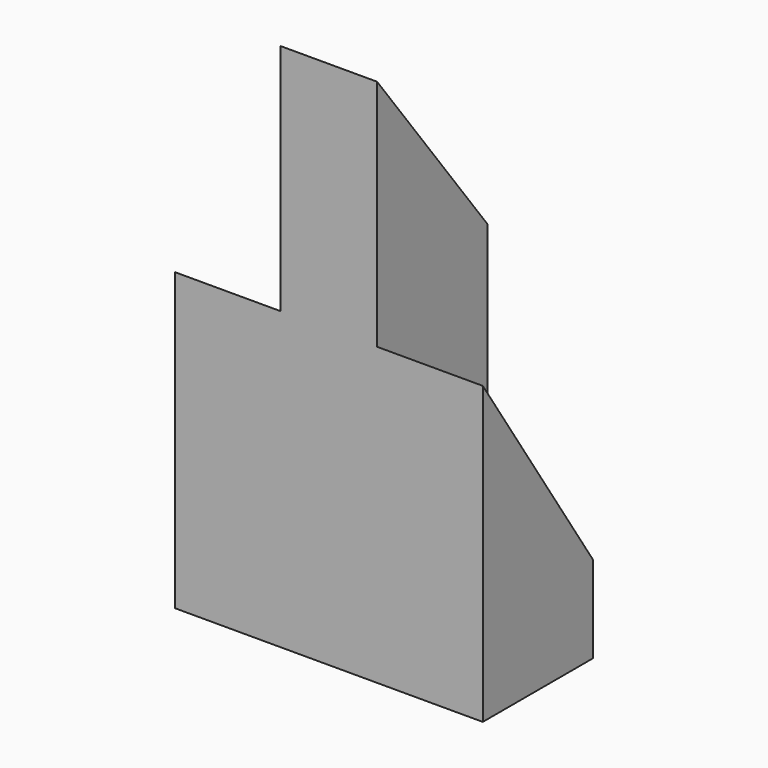
from build123d import *

# Parameters (mm, degrees)
F0_W      = 44.45
F0_H      = 38.1
F1_DEPTH  = 25.4
F2_DEPTH  = 56.388
F3_DEPTH  = 85.09
F6_DEPTH  = 29.21
F7_DEPTH  = 29.21
F8_DEPTH  = 64.516
F10_DEPTH = 25.4
F11_DEPTH = 25.4


with BuildPart() as f1:
    # F0 (on Top) → F1 (new body)
    with BuildSketch(Plane.XY):
        with Locations((-37.1782257403, 19.05)):
            Rectangle(F0_W, F0_H)
    extrude(amount=F1_DEPTH)

    # F2 (add): a face of the model
    f2_faces = [f1.faces().sort_by_distance(p)[0] for p in [
        (-37.1782257403, 19.05, 0),
    ]]
    extrude(f2_faces, amount=F2_DEPTH)

    # F3 (add): a face of the model
    f3_faces = [f1.faces().sort_by_distance(p)[0] for p in [
        (-59.4032257403, 19.05, -15.494),
    ]]
    extrude(f3_faces, amount=-F3_DEPTH)

    # F5 (on face) → F6 (cut)
    with BuildSketch(Plane.YZ.offset(25.6867742597)):
        Polygon((0, 25.4), (38.1, -32.4071533978), (38.1, 25.4), align=None)
    extrude(amount=-F6_DEPTH, mode=Mode.SUBTRACT)

    # F4 (on face) → F7 (cut)
    with BuildSketch(Plane(origin=(-59.4032257403, 0, 0), x_dir=(0, -1, 0), z_dir=(-1, 0, 0))):
        Polygon((-38.1, 25.4), (-38.1, -32.3631092906), (0, 25.4), align=None)
    extrude(amount=-F7_DEPTH, mode=Mode.SUBTRACT)

    # F8 (add): a face of the model
    f8_faces = [f1.faces().sort_by_distance(p)[0] for p in [
        (-16.8582257403, 19.05, 25.4),
    ]]
    extrude(f8_faces, amount=F8_DEPTH)

    # F9 (on face) → F10 (cut)
    with BuildSketch(Plane(origin=(-30.1932257403, 0, 0), x_dir=(0, -1, 0), z_dir=(-1, 0, 0))):
        Polygon((-38.1, 89.916), (-38.1, 39.8104563355), (0, 89.916), align=None)
    extrude(amount=-F10_DEPTH, mode=Mode.SUBTRACT)

    # F11 (cut): a face of the model
    f11_faces = [f1.faces().sort_by_distance(p)[0] for p in [
        (-4.7932257403, 25.4, 73.2141521118),
    ]]
    extrude(f11_faces, amount=-F11_DEPTH, mode=Mode.SUBTRACT)


solid = f1.part
